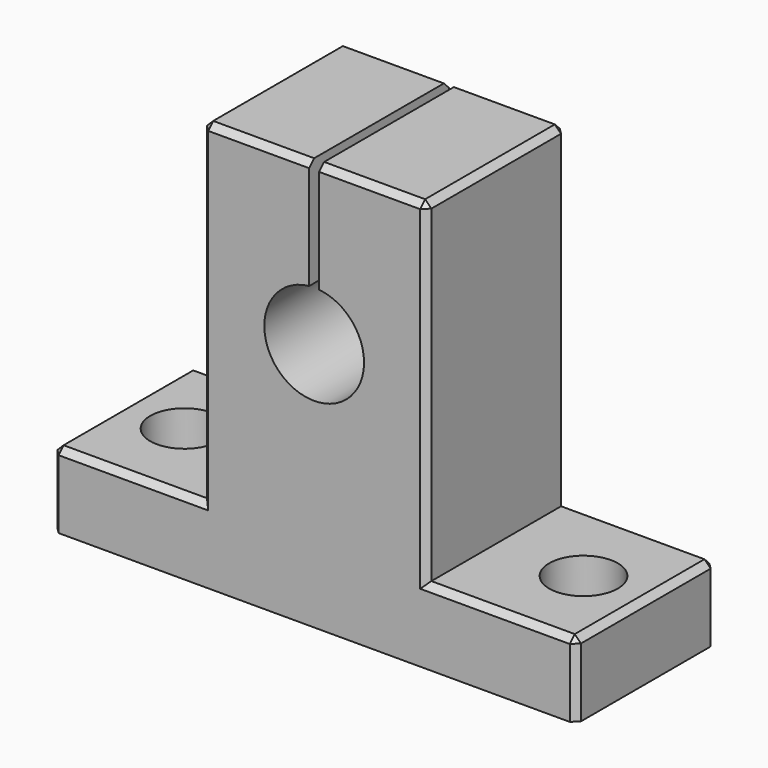
from build123d import *

# Parameters (mm, degrees)
F1_DEPTH = 14
F2_R     = 2.75
F3_DEPTH = 6
F4_SIZE  = 0.5


with BuildPart() as f1:
    # F0 (on Front) → F1 (new body)
    with BuildSketch(Plane.XZ):
        with BuildLine():
            Line((-21, -10.4), (-21, -16.4))
            Line((-21, -16.4), (21, -16.4))
            Line((21, -16.4), (21, -10.4))
            Line((21, -10.4), (9, -10.4))
            Line((9, -10.4), (9, 16.4))
            Line((9, 16.4), (0.4, 16.4))
            Line((0.4, 16.4), (0.4, 7.5799497484))
            ThreePointArc((0.4, 7.5799497484), (2.9664793948, 6.283281573), (4, 3.6))
            ThreePointArc((4, 3.6), (-2.683281573, 0.6335206052), (-0.4, 7.5799497484))
            Line((-0.4, 7.5799497484), (-0.4, 16.4))
            Line((-0.4, 16.4), (-9, 16.4))
            Line((-9, 16.4), (-9, -10.4))
            Line((-9, -10.4), (-21, -10.4))
        make_face()
    extrude(amount=F1_DEPTH)

    # F2 (on face) → F3 (cut)
    with BuildSketch(Plane(origin=(0, 0, -16.4), x_dir=(1, 0, 0), z_dir=(0, 0, -1))):
        with Locations((-16, 7)):
            Circle(F2_R)
        with Locations((16, 7)):
            Circle(F2_R)
    extrude(amount=-F3_DEPTH, mode=Mode.SUBTRACT)

    # F4
    f4_edges = [f1.edges().sort_by_distance(p)[0] for p in [
        (9, -7, 16.4),
        (-4.7, -14, 16.4),
        (-4.7, 0, 16.4),
        (-9, -7, 16.4),
        (9, -14, 3),
        (9, 0, 3),
        (15, 0, -10.4),
        (15, -14, -10.4),
        (21, -7, -10.4),
        (21, -14, -13.4),
        (21, 0, -13.4),
        (-9, -14, 3),
        (-15, -14, -10.4),
        (-21, -14, -13.4),
        (-21, -7, -10.4),
        (-9, 0, 3),
        (-15, 0, -10.4),
        (-21, 0, -13.4),
        (4.7, 0, 16.4),
        (4.7, -14, 16.4),
    ]]
    chamfer(f4_edges, length=F4_SIZE)


solid = f1.part
